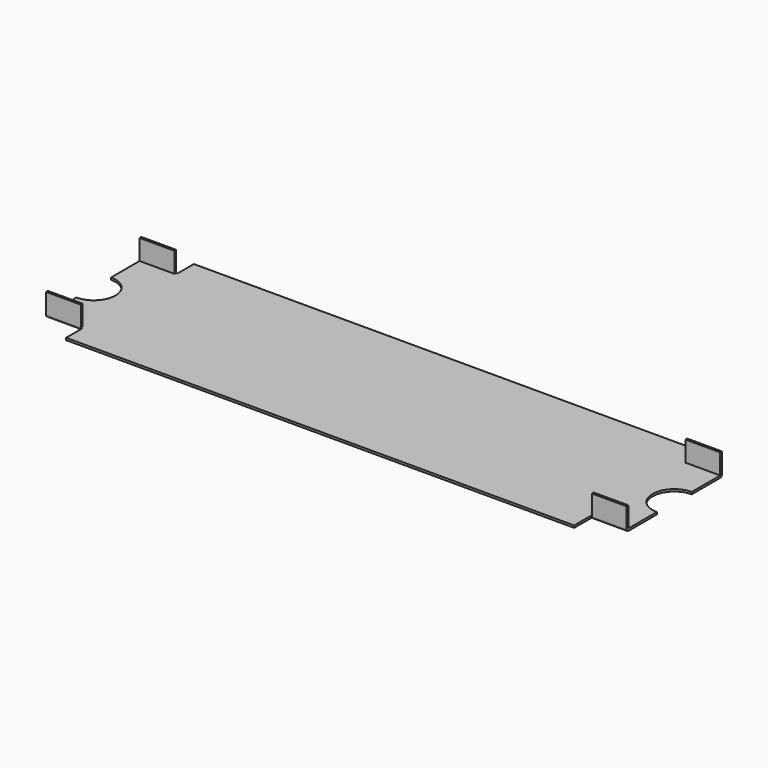
from build123d import *

# Parameters (mm, degrees)
F1_DEPTH = 1.5
F3_W     = 24
F3_H     = 1.5
F4_DEPTH = 14
F5_R     = 1.49999


# Not quite as in the source:
# - a fillet or chamfer is up to 0.001 mm smaller than in the source, because OpenCascade refuses the exact size


with BuildPart() as f1:
    # F0 (on Top) → F1 (new body)
    with BuildSketch(Plane.XY):
        with BuildLine():
            Line((375, 14), (25, 14))
            Line((25, 14), (25, 0))
            Line((25, 0), (0, 0))
            Line((0, 0), (0, -26))
            ThreePointArc((0, -26), (15, -41), (0, -56))
            Line((0, -56), (0, -82))
            Line((0, -82), (25, -82))
            Line((25, -82), (25, -96))
            Line((25, -96), (375, -96))
            Line((375, -96), (375, -82))
            Line((375, -82), (400, -82))
            Line((400, -82), (400, -56))
            ThreePointArc((400, -56), (385, -41), (400, -26))
            Line((400, -26), (400, 0))
            Line((400, 0), (375, 0))
            Line((375, 0), (375, 14))
        make_face()
    extrude(amount=F1_DEPTH)

    # F3 (on face) → F4 (join)
    with BuildSketch(Plane.XY.offset(1.5)):
        with Locations((12, -0.75)):
            Rectangle(F3_W, F3_H)
        with Locations((388, -0.75)):
            Rectangle(F3_W, F3_H)
        with Locations((12, -81.25)):
            Rectangle(F3_W, F3_H)
        with Locations((388, -81.25)):
            Rectangle(F3_W, F3_H)
    extrude(amount=F4_DEPTH)

    # F5 (radius 1.5 in the source; OpenCascade refuses exactly that, so slightly less here)
    f5_edges = [f1.edges().sort_by_distance(p)[0] for p in [
        (12.5, 0, 0),
        (12.5, -82, 0),
        (387.5, -82, 0),
        (387.5, 0, 0),
    ]]
    fillet(f5_edges, radius=F5_R)


solid = f1.part
